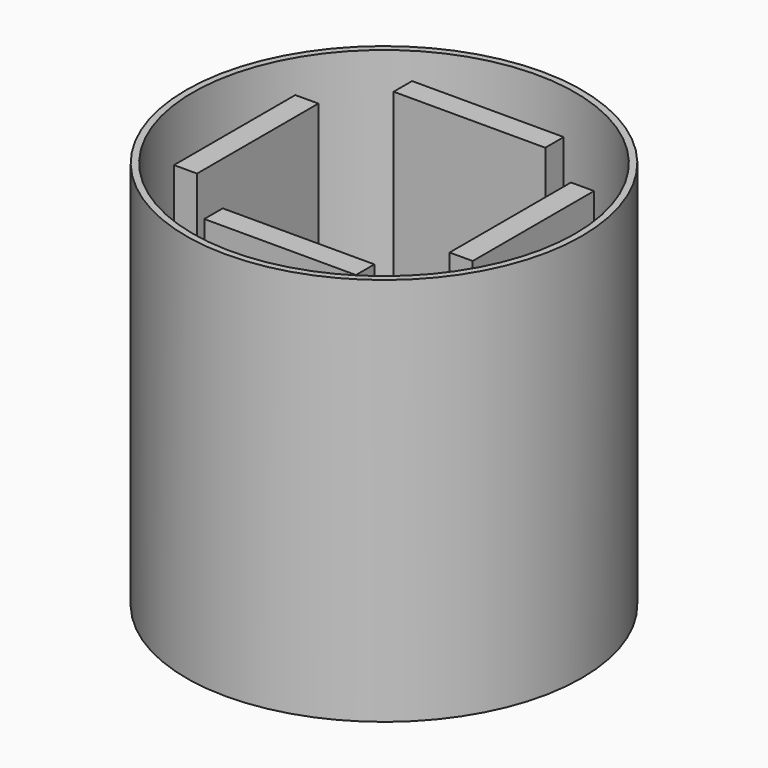
from build123d import *

# Parameters (mm, degrees)
F0_R     = 300
F0_R_2   = 290
F0_R_3   = 12.5
F1_DEPTH = 10
F2_DEPTH = 590
F5_START = 100
F4_W     = 35
F4_H     = 230
F5_DEPTH = 460
F6_COUNT = 4


# Not quite as in the source:
# - the program builds the solid bodies; features that only make, move or delete a surface that nothing else refers to are left out


with BuildPart() as f1:
    # F0 (on Top) → F1 (new body)
    with BuildSketch(Plane.XY):
        Circle(F0_R)
        Circle(F0_R_2, mode=Mode.SUBTRACT)
        Circle(F0_R_2)
        Circle(F0_R_3, mode=Mode.SUBTRACT)
    extrude(amount=F1_DEPTH)

    # F0 (on Top) → F2 (join)
    with BuildSketch(Plane.XY):
        Circle(F0_R)
        Circle(F0_R_2, mode=Mode.SUBTRACT)
    extrude(amount=F2_DEPTH)


with BuildPart() as f5:
    # F4 (on face) → F5 (new body)
    with BuildSketch(Plane.XY.offset(10).offset(F5_START)):
        with Locations((-197.5, -14.4088214636)):
            Rectangle(F4_W, F4_H)
    extrude(amount=F5_DEPTH)


with BuildPart() as f6_1:
    # F6: instance of F5
    add(f5.part.rotate(Axis((0, 0, 0), (0, 0, 1)), 1 * 360 / F6_COUNT))


with BuildPart() as f6_2:
    # F6: instance of F5
    add(f5.part.rotate(Axis((0, 0, 0), (0, 0, 1)), 2 * 360 / F6_COUNT))


with BuildPart() as f6_3:
    # F6: instance of F5
    add(f5.part.rotate(Axis((0, 0, 0), (0, 0, 1)), 3 * 360 / F6_COUNT))


solid = Compound([f1.part, f5.part, f6_1.part, f6_2.part, f6_3.part])
